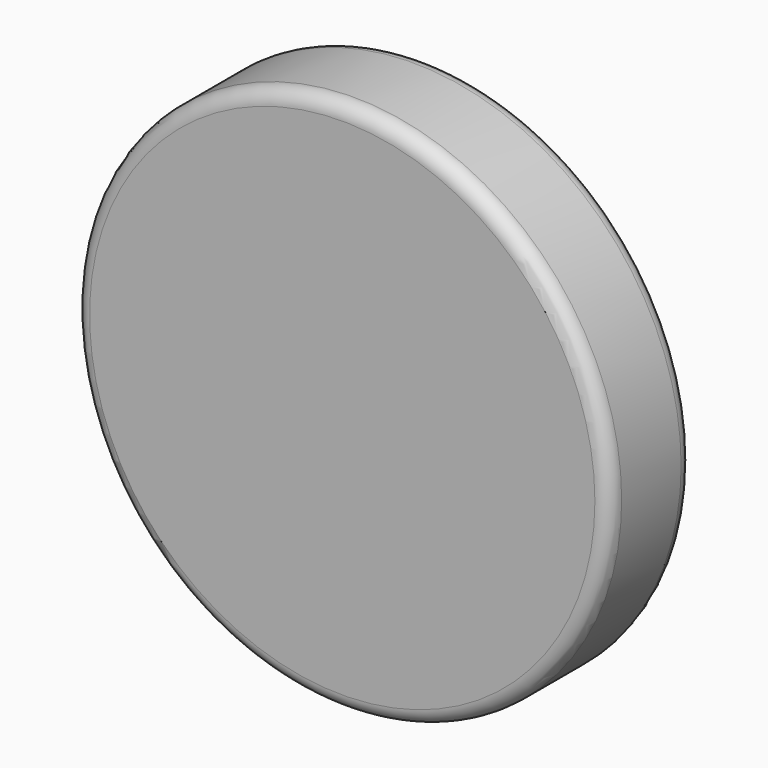
from build123d import *

# Parameters (mm, degrees)
F0_R     = 18
F0_R_2   = 13.6738896343
F2_DEPTH = 7
F1_R     = 13.7073607276
F3_DEPTH = 8
F4_R     = 1


# Not quite as in the source:
# - a fillet or chamfer that OpenCascade refuses, or shapes differently, is made with other operations: its cross-section is extruded or revolved along the edge and cut away or added


with BuildPart() as f2:
    # F0 (on Front) → F2 (new body)
    with BuildSketch(Plane.XZ):
        Circle(F0_R)
        Circle(F0_R_2, mode=Mode.SUBTRACT)
    extrude(amount=-F2_DEPTH)

    # F1 (on Front) → F3 (join)
    with BuildSketch(Plane.XZ):
        Circle(F1_R)
    extrude(amount=-F3_DEPTH)

    # F4
    f4_edges = [f2.edges().sort_by_distance(p)[0] for p in [
        (18, 3.5, 0),
        (-18, 0, 0),
        (-18, 7, 0),
    ]]
    fillet(f4_edges, radius=F4_R)

    # F5: fillet of radius 90 on 1 edges, made by hand

    # F5_s1 → F5_t2 (revolve, cut)
    with BuildSketch(Plane.XY):
        with BuildLine():
            ThreePointArc((13.7073607276, 7), (7.0364764999, 7.7496518099), (0.3282725674, 8))
            Line((0.3282725674, 8), (13.7073607276, 8))
            Line((13.7073607276, 8), (13.7073607276, 7))
        make_face()
    revolve(axis=Axis((0, 8, 0), (0, -1, 0)), mode=Mode.SUBTRACT)


solid = f2.part
